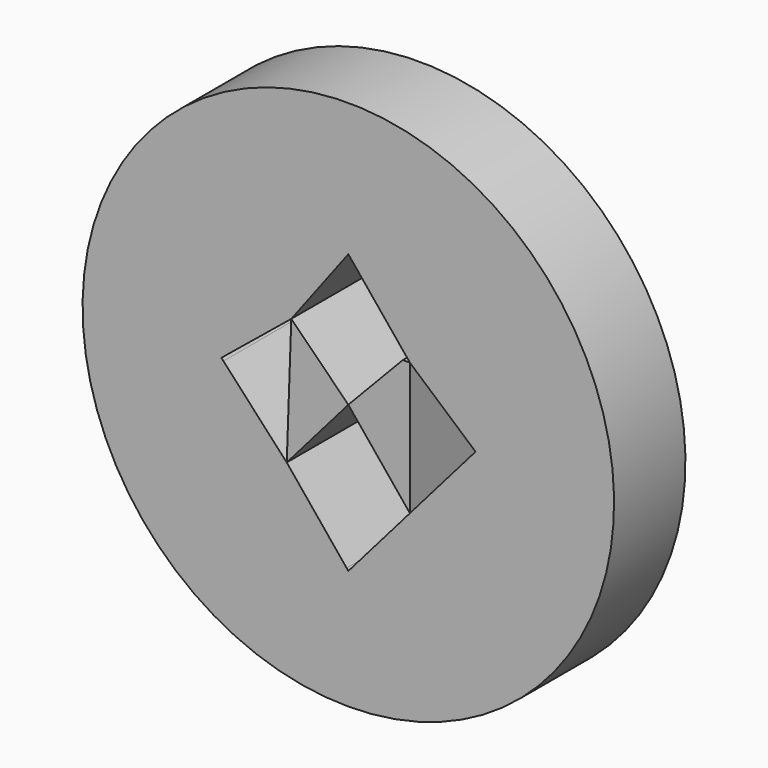
from build123d import *

# Parameters (mm, degrees)
F1_DEPTH = 25.4


with BuildPart() as f1:
    # F0 (on Front) → F1 (new body)
    with BuildSketch(Plane.XZ):
        with BuildLine():
            Line((36.0940568046, 37.8100693834), (75.7017228123, 0))
            ThreePointArc((75.7017228123, 0), (0, 75.7017228123), (-75.7017228123, 0))
            Line((-75.7017228123, 0), (-1.7577517696, 73.9439710427))
            Line((-1.7577517696, 73.9439710427), (36.0940568046, 37.8100693834))
        make_face()
        Polygon((34.0044190793, -41.6973037331), (75.7017228123, 0), (36.0940568046, 37.8100693834), (35.1256847707, 0.9650623831), (36.2361905576, 0), (35.0648969253, -1.3478179023), align=None)
        with BuildLine():
            ThreePointArc((0, -75.7017228123), (53.5292015481, -53.5292015481), (75.7017228123, 0))
            Line((75.7017228123, 0), (34.0044190793, -41.6973037331))
            Line((34.0044190793, -41.6973037331), (0, -75.7017228123))
        make_face()
        with BuildLine():
            Line((-35.1984994172, -40.5032233952), (-75.7017228123, 0))
            ThreePointArc((-75.7017228123, 0), (-53.5292015481, -53.5292015481), (0, -75.7017228123))
            Line((0, -75.7017228123), (-35.1984994172, -40.5032233952))
        make_face()
        Polygon((-1.7577517696, 73.9439710427), (-75.7017228123, 0), (-35.1984994172, -40.5032233952), (-35.5822025801, -0.6328943901), (-36.1661069663, 0), (-35.5927929278, 0.4675412817), (-35.9341153342, 35.9341153342), (-37.8100693834, 37.8100693834), (36.0940568046, 37.8100693834), align=None)
        Polygon((-35.1984994172, -40.5032233952), (0, -75.7017228123), (34.0044190793, -41.6973037331), (0.5023601674, -41.1192334624), (0, -41.6973037331), (-0.4853180091, -41.1021913041), align=None)
        Polygon((35.1256847707, 0.9650623831), (36.0940568046, 37.8100693834), (16.6052143863, 17.3946727981), (17.5424247587, 16.2454355338), align=None)
        Polygon((16.6052143863, 17.3946727981), (36.0940568046, 37.8100693834), (-37.8100693834, 37.8100693834), (-35.9341153342, 35.9341153342), (-16.2454355338, 16.2454355338), (0, 37.7565165398), align=None)
        Polygon((0.5023601674, -41.1192334624), (34.0044190793, -41.6973037331), (17.5424247587, -21.511081006), align=None)
        Polygon((17.5424247587, -21.511081006), (34.0044190793, -41.6973037331), (35.0648969253, -1.3478179023), align=None)
        Polygon((-35.5822025801, -0.6328943901), (-35.1984994172, -40.5032233952), (-17.5424247587, -20.1862227271), align=None)
        Polygon((-17.5424247587, -20.1862227271), (-35.1984994172, -40.5032233952), (-0.4853180091, -41.1021913041), align=None)
        Polygon((-16.2454355338, 16.2454355338), (-35.9341153342, 35.9341153342), (-35.5927929278, 0.4675412817), align=None)
    extrude(amount=F1_DEPTH)


with BuildPart() as f1b:
    # F0 (on Front) → F1, piece 2 (new body)
    with BuildSketch(Plane.XZ):
        Polygon((0, 0), (17.5424247587, -21.511081006), (17.5424247587, 16.2454355338), (15.5081353336, 16.2454355338), align=None)
    extrude(amount=F1_DEPTH)


with BuildPart() as f1c:
    # F0 (on Front) → F1, piece 3 (new body)
    with BuildSketch(Plane.XZ):
        Polygon((-16.2454355338, 16.2454355338), (-17.5424247587, -20.1862227271), (0, 0), align=None)
    extrude(amount=F1_DEPTH)


solid = Compound([f1.part, f1b.part, f1c.part])
